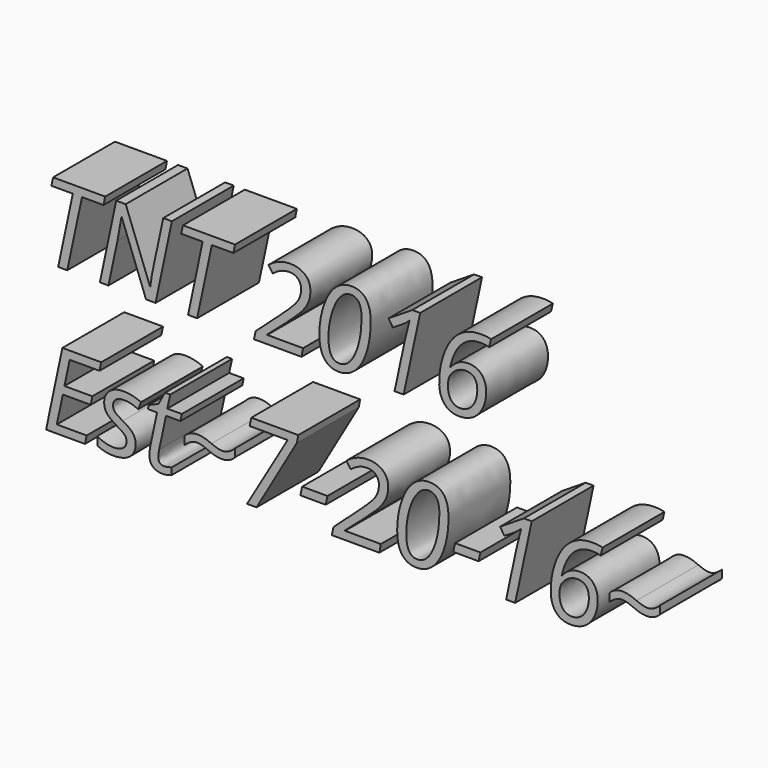
from build123d import *

# Parameters (mm, degrees)
F0_TEXT_SIZE = 35.5456386589
F1_DEPTH     = 25.4


# Not quite as in the source:
# - Text() gives the source's letters only with a copy of the font that has no kerning and outlines rounded to 1/6400 em; it was checked with that copy


with BuildPart() as f1:
    # F0 (on Front) → F1 (new body)
    with BuildSketch(Plane.XZ):
        with Locations((-35.157866776, -7.6261553913)):
            Text('TNT 2016', F0_TEXT_SIZE, font='Open Sans', font_style=FontStyle.ITALIC, text_align=(TextAlign.LEFT, TextAlign.BOTTOM))
        with Locations((-35.157866776, -55.9682239675)):
            Text('Est~7-20-16~', F0_TEXT_SIZE, font='Open Sans', font_style=FontStyle.ITALIC, text_align=(TextAlign.LEFT, TextAlign.BOTTOM))
    extrude(amount=F1_DEPTH)


solid = f1.part
